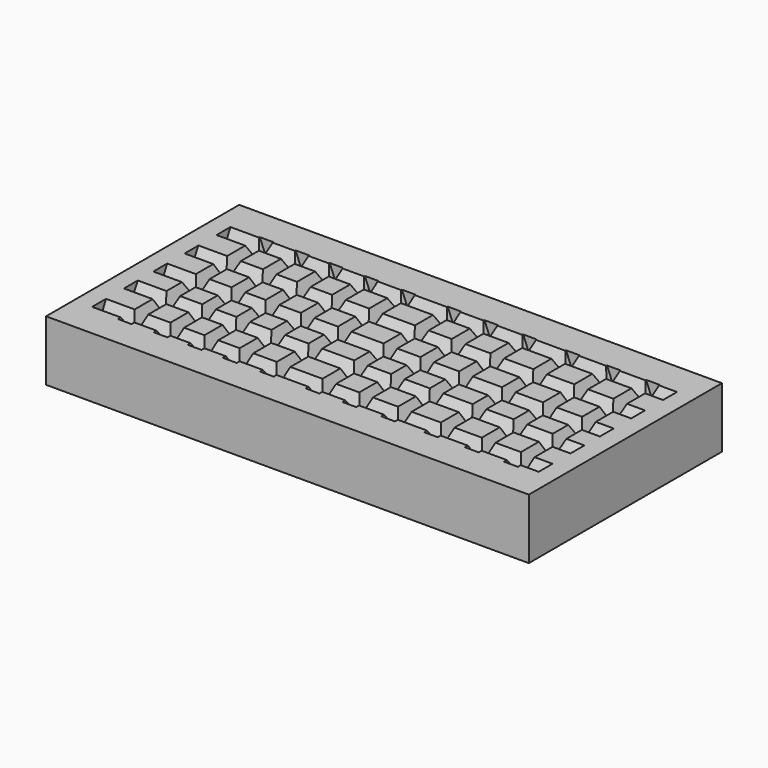
from build123d import *

# Parameters (mm, degrees)
F0_W          = 40
F0_H          = 20
F1_DEPTH      = 5
F3_DEPTH      = 18.5
F3_DEPTH_BACK = 18.5
F5_START      = -2.6
F5_DEPTH      = 14.7


with BuildPart() as f1:
    # F0 (on Top) → F1 (new body)
    with BuildSketch(Plane.XY):
        Rectangle(F0_W, F0_H)
    extrude(amount=F1_DEPTH)

    # F2 (on Right) → F3 (cut, two sides)
    with BuildSketch(Plane.YZ) as f3_sk:
        Polygon((0.3706877469, 5.1759975031), (-0.3706877469, 5.1759975031), (-0.8703563362, 5.1759975031), (0, 3.6660050973), (0.7561275852, 5.1759975031), align=None)
        Polygon((4.0111204144, 5.1759975031), (3.511451825, 5.1759975031), (2.7700763312, 5.1759975031), (2.3846364929, 5.1759975031), (3.1407640781, 3.6660050973), align=None)
        Polygon((6.5501930658, 3.6660050973), (7.306320651, 5.1759975031), (6.9208808127, 5.1759975031), (6.1795053189, 5.1759975031), (5.6798367295, 5.1759975031), align=None)
        Polygon((-3.1407640781, 3.6660050973), (-2.2704077419, 5.1759975031), (-2.7700763312, 5.1759975031), (-3.511451825, 5.1759975031), (-3.8968916633, 5.1759975031), align=None)
        Polygon((-6.3353183214, 3.6660050973), (-5.5791907362, 5.1759975031), (-5.9646305745, 5.1759975031), (-6.7060060683, 5.1759975031), (-7.2056746576, 5.1759975031), align=None)
    extrude(amount=-F3_DEPTH, mode=Mode.SUBTRACT)
    extrude(f3_sk.sketch, amount=F3_DEPTH_BACK, mode=Mode.SUBTRACT)

    # F4 (on face) → F5 (cut)
    with BuildSketch(Plane.XZ.offset(10).offset(F5_START)):
        Polygon((0.6511597122, 5.2109442782), (0, 5.2109442782), (-0.6511597122, 5.2109442782), (0, 3.59428511), align=None)
        Polygon((-3.7887066137, 3.59428511), (-3.1375469015, 5.2109442782), (-3.7887066137, 5.2109442782), (-4.4398663259, 5.2109442782), align=None)
        Polygon((-7.5088410332, 5.2109442782), (-6.857681321, 3.59428511), (-6.2065216088, 5.2109442782), (-6.857681321, 5.2109442782), align=None)
        Polygon((-9.7715433221, 3.59428511), (-9.1203836099, 5.2109442782), (-9.7715433221, 5.2109442782), (-10.4227030343, 5.2109442782), align=None)
        Polygon((-13.2457284881, 5.2109442782), (-12.594568776, 3.59428511), (-11.9434090638, 5.2109442782), (-12.594568776, 5.2109442782), align=None)
        Polygon((-15.5610654037, 3.59428511), (-14.9099056916, 5.2109442782), (-15.5610654037, 5.2109442782), (-16.2122251159, 5.2109442782), align=None)
        Polygon((2.4007019428, 5.2109442782), (3.051861655, 3.59428511), (3.7030213672, 5.2109442782), (3.051861655, 5.2109442782), align=None)
        Polygon((6.2590357848, 5.2109442782), (5.6078760726, 5.2109442782), (6.2590357848, 3.59428511), (6.9101954969, 5.2109442782), align=None)
        Polygon((9.1604591188, 5.2109442782), (9.811618831, 3.59428511), (10.4627785432, 5.2109442782), (9.811618831, 5.2109442782), align=None)
        Polygon((13.2065662183, 5.2109442782), (12.5554065061, 5.2109442782), (13.2065662183, 3.59428511), (13.8577259305, 5.2109442782), align=None)
        Polygon((15.795035365, 5.2109442782), (16.4461950772, 3.59428511), (17.0973547893, 5.2109442782), (16.4461950772, 5.2109442782), align=None)
    extrude(amount=-F5_DEPTH, mode=Mode.SUBTRACT)


solid = f1.part
